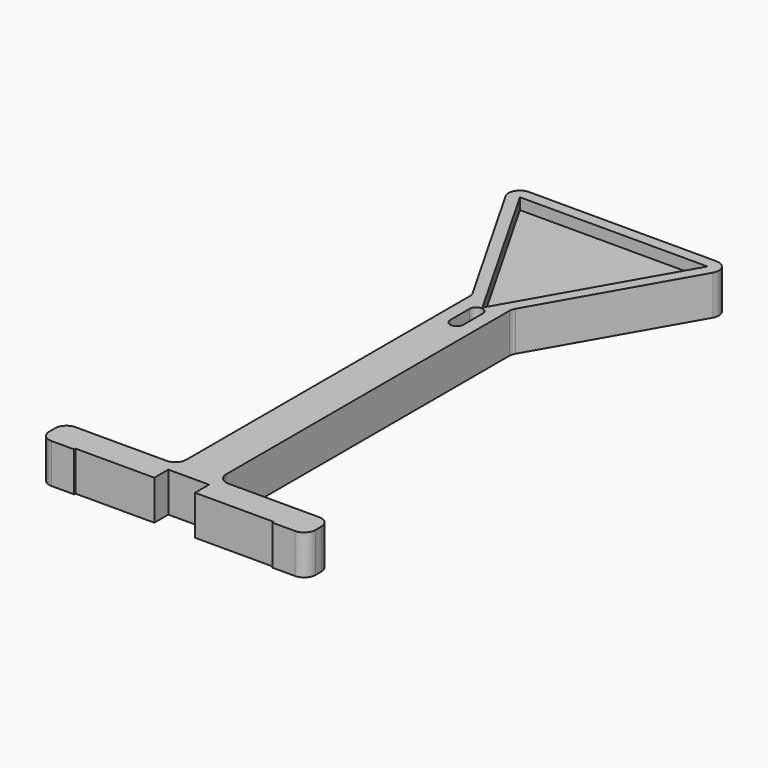
from build123d import *

# Parameters (mm, degrees)
F0_W     = 6
F0_H     = 0.3
F1_DEPTH = 7
F3_DEPTH = 2
F4_R     = 2
F5_W     = 2.3
F5_H     = 4.3
F6_DEPTH = 3.5


# Not quite as in the source:
# - a feature names something its author has since deleted; it is built from what else it names


with BuildPart() as f1:
    # F0 (on Top) → F1 (new body)
    with BuildSketch(Plane.XY):
        Polygon((0, -7), (-3.5, -0.875), (-3.5, -65.875), (-23.5, -65.875), (-23.5, -70.875), (-17.5, -70.875), (-3.6, -70.875), (-3.6, -67.775), (3.6, -67.775), (3.6, -70.875), (17.5, -70.875), (23.5, -70.875), (23.5, -65.875), (3.5, -65.875), (3.5, -0.875), align=None)
        with Locations((-20.5, -71.025)):
            Rectangle(F0_W, F0_H)
        with Locations((20.5, -71.025)):
            Rectangle(F0_W, F0_H)
        Polygon((-20, 28), (-3.5, -0.875), (0, -7), (3.5, -0.875), (20, 28), align=None)
    extrude(amount=F1_DEPTH)

    # F2 (on face) → F3 (cut)
    with BuildSketch(Plane.XY.offset(7)):
        Polygon((16.5536406433, 26), (-16.5536406433, 26), (0, -2.9688711259), align=None)
    extrude(amount=-F3_DEPTH, mode=Mode.SUBTRACT)

    # F4
    f4_edges = [f1.edges().sort_by_distance(p)[0] for p in [
        (3.5, -65.875, 3.5),
        (-3.5, -65.875, 3.5),
        (-23.5, -65.875, 3.5),
        (23.5, -65.875, 3.5),
        (-23.5, -71.175, 3.5),
        (23.5, -71.175, 3.5),
        (-20, 28, 3.5),
        (20, 28, 3.5),
        (-3.5, -0.875, 3.5),
        (3.5, -0.875, 3.5),
    ]]
    fillet(f4_edges, radius=F4_R)

    # F5 (on face) → F6 (cut)
    with BuildSketch(Plane.XY.offset(7)):
        with BuildLine():
            ThreePointArc((-1.15, -8.6188711259), (0, -9.7688711259), (1.15, -8.6188711259))
            Line((1.15, -8.6188711259), (-1.15, -8.6188711259))
        make_face()
        with Locations((0, -6.4688711259)):
            Rectangle(F5_W, F5_H)
        with BuildLine():
            Line((-1.15, -4.3188711259), (1.15, -4.3188711259))
            ThreePointArc((1.15, -4.3188711259), (0, -3.1688711259), (-1.15, -4.3188711259))
        make_face()
    extrude(amount=-F6_DEPTH, mode=Mode.SUBTRACT)


solid = f1.part
